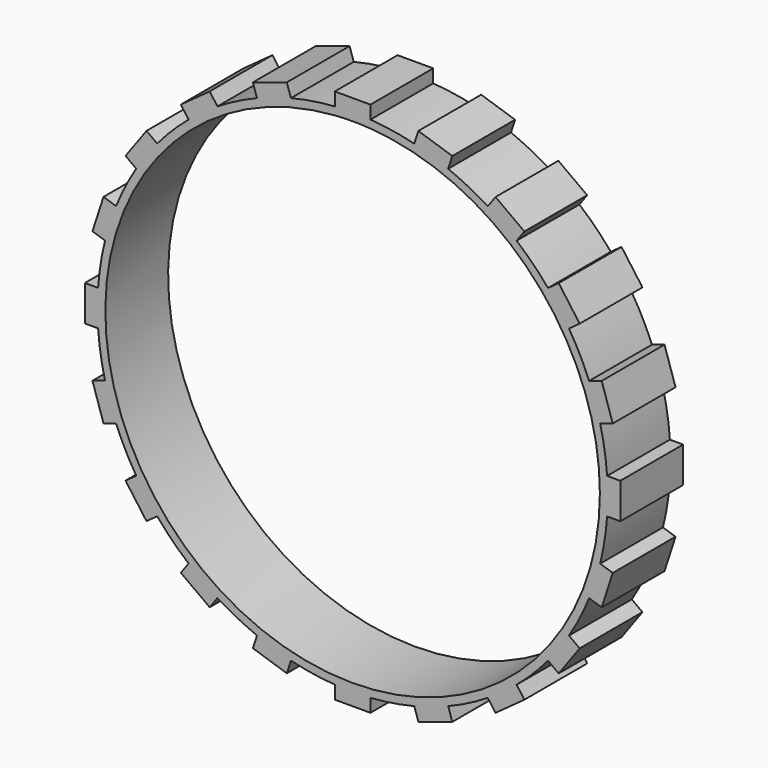
from build123d import *

# Parameters (mm, degrees)
F1_DEPTH = 10.16


with BuildPart() as f1:
    # F0 (on Front) → F1 (new body)
    with BuildSketch(Plane.XZ):
        with BuildLine():
            ThreePointArc((32.9392262703, -2.3081968538), (32.9998003891, -1.1548048657), (33.02, 0))
            ThreePointArc((33.02, 0), (32.9998003891, 1.1548048657), (32.9392262703, 2.3081968538))
            ThreePointArc((32.9392262703, 2.3081968538), (32.6134690065, 5.1654660356), (32.0403378403, 7.9835550403))
            ThreePointArc((32.0403378403, 7.9835550403), (31.4038861681, 10.2037411543), (30.6137937319, 12.3740063578))
            ThreePointArc((30.6137937319, 12.3740063578), (29.4210354287, 14.9907663014), (28.0051179043, 17.4938209425))
            ThreePointArc((28.0051179043, 17.4938209425), (26.7137411543, 19.4086690307), (25.2916697641, 21.2285619047))
            ThreePointArc((25.2916697641, 21.2285619047), (23.3486659148, 23.3486659148), (21.2285619047, 25.2916697641))
            ThreePointArc((21.2285619047, 25.2916697641), (19.4086690307, 26.7137411543), (17.4938209425, 28.0051179043))
            ThreePointArc((17.4938209425, 28.0051179043), (14.9907663014, 29.4210354287), (12.3740063578, 30.6137937319))
            ThreePointArc((12.3740063578, 30.6137937319), (10.2037411543, 31.4038861681), (7.9835550403, 32.0403378403))
            ThreePointArc((7.9835550403, 32.0403378403), (5.1654660356, 32.6134690065), (2.3081968538, 32.9392262703))
            ThreePointArc((2.3081968538, 32.9392262703), (0, 33.02), (-2.3081968538, 32.9392262703))
            ThreePointArc((-2.3081968538, 32.9392262703), (-5.1654660356, 32.6134690065), (-7.9835550403, 32.0403378403))
            ThreePointArc((-7.9835550403, 32.0403378403), (-10.2037411543, 31.4038861681), (-12.3740063578, 30.6137937319))
            ThreePointArc((-12.3740063578, 30.6137937319), (-14.9907663014, 29.4210354287), (-17.4938209425, 28.0051179043))
            ThreePointArc((-17.4938209425, 28.0051179043), (-19.4086690307, 26.7137411543), (-21.2285619047, 25.2916697641))
            ThreePointArc((-21.2285619047, 25.2916697641), (-23.3486659148, 23.3486659148), (-25.2916697641, 21.2285619047))
            ThreePointArc((-25.2916697641, 21.2285619047), (-26.7137411543, 19.4086690307), (-28.0051179043, 17.4938209425))
            ThreePointArc((-28.0051179043, 17.4938209425), (-29.4210354287, 14.9907663014), (-30.6137937319, 12.3740063578))
            ThreePointArc((-30.6137937319, 12.3740063578), (-31.4038861681, 10.2037411543), (-32.0403378403, 7.9835550403))
            ThreePointArc((-32.0403378403, 7.9835550403), (-32.6134690065, 5.1654660356), (-32.9392262703, 2.3081968538))
            ThreePointArc((-32.9392262703, 2.3081968538), (-33.02, 0), (-32.9392262703, -2.3081968538))
            ThreePointArc((-32.9392262703, -2.3081968538), (-32.6134690065, -5.1654660356), (-32.0403378403, -7.9835550403))
            ThreePointArc((-32.0403378403, -7.9835550403), (-31.4038861681, -10.2037411543), (-30.6137937319, -12.3740063578))
            ThreePointArc((-30.6137937319, -12.3740063578), (-29.4210354287, -14.9907663014), (-28.0051179043, -17.4938209425))
            ThreePointArc((-28.0051179043, -17.4938209425), (-26.7137411543, -19.4086690307), (-25.2916697641, -21.2285619047))
            ThreePointArc((-25.2916697641, -21.2285619047), (-23.3486659148, -23.3486659148), (-21.2285619047, -25.2916697641))
            ThreePointArc((-21.2285619047, -25.2916697641), (-19.4086690307, -26.7137411543), (-17.4938209425, -28.0051179043))
            ThreePointArc((-17.4938209425, -28.0051179043), (-14.9907663014, -29.4210354287), (-12.3740063578, -30.6137937319))
            ThreePointArc((-12.3740063578, -30.6137937319), (-10.2037411543, -31.4038861681), (-7.9835550403, -32.0403378403))
            ThreePointArc((-7.9835550403, -32.0403378403), (-5.1654660356, -32.6134690065), (-2.3081968538, -32.9392262703))
            ThreePointArc((-2.3081968538, -32.9392262703), (0, -33.02), (2.3081968538, -32.9392262703))
            ThreePointArc((2.3081968538, -32.9392262703), (5.1654660356, -32.6134690065), (7.9835550403, -32.0403378403))
            ThreePointArc((7.9835550403, -32.0403378403), (10.2037411543, -31.4038861681), (12.3740063578, -30.6137937319))
            ThreePointArc((12.3740063578, -30.6137937319), (14.9907663014, -29.4210354287), (17.4938209425, -28.0051179043))
            ThreePointArc((17.4938209425, -28.0051179043), (19.4086690307, -26.7137411543), (21.2285619047, -25.2916697641))
            ThreePointArc((21.2285619047, -25.2916697641), (23.3486659148, -23.3486659148), (25.2916697641, -21.2285619047))
            ThreePointArc((25.2916697641, -21.2285619047), (26.7137411543, -19.4086690307), (28.0051179043, -17.4938209425))
            ThreePointArc((28.0051179043, -17.4938209425), (29.4210354287, -14.9907663014), (30.6137937319, -12.3740063578))
            ThreePointArc((30.6137937319, -12.3740063578), (31.4038861681, -10.2037411543), (32.0403378403, -7.9835550403))
            ThreePointArc((32.0403378403, -7.9835550403), (32.6134690065, -5.1654660356), (32.9392262703, -2.3081968538))
        make_face()
        with BuildLine():
            ThreePointArc((2.3081968538, 31.9206554332), (23.4321098934, 21.7989046042), (32.004, 0))
            ThreePointArc((32.004, 0), (-21.7989046042, -23.4321098934), (-2.3081968538, 31.9206554332))
            ThreePointArc((-2.3081968538, 31.9206554332), (0, 32.004), (2.3081968538, 31.9206554332))
        make_face(mode=Mode.SUBTRACT)
        with BuildLine():
            ThreePointArc((32.9392262703, 2.3081968538), (32.9998003891, 1.1548048657), (33.02, 0))
            ThreePointArc((33.02, 0), (32.9998003891, -1.1548048657), (32.9392262703, -2.3081968538))
            Line((32.9392262703, -2.3081968538), (34.6495732665, -2.3081968538))
            Line((34.6495732665, -2.3081968538), (34.6495732665, 2.3081968538))
            Line((34.6495732665, 2.3081968538), (32.9392262703, 2.3081968538))
        make_face()
        with BuildLine():
            ThreePointArc((30.6137937319, 12.3740063578), (31.4038861681, 10.2037411543), (32.0403378403, 7.9835550403))
            Line((32.0403378403, 7.9835550403), (33.6669744962, 8.5120813284))
            Line((33.6669744962, 8.5120813284), (32.2404303878, 12.9025326459))
            Line((32.2404303878, 12.9025326459), (30.6137937319, 12.3740063578))
        make_face()
        with BuildLine():
            Line((33.6669744962, -8.5120813284), (32.0403378403, -7.9835550403))
            ThreePointArc((32.0403378403, -7.9835550403), (31.4038861681, -10.2037411543), (30.6137937319, -12.3740063578))
            Line((30.6137937319, -12.3740063578), (32.2404303878, -12.9025326459))
            Line((32.2404303878, -12.9025326459), (33.6669744962, -8.5120813284))
        make_face()
        with BuildLine():
            ThreePointArc((25.2916697641, 21.2285619047), (26.7137411543, 19.4086690307), (28.0051179043, 17.4938209425))
            Line((28.0051179043, 17.4938209425), (29.3888176905, 18.4991376832))
            Line((29.3888176905, 18.4991376832), (26.6753695504, 22.2338786454))
            Line((26.6753695504, 22.2338786454), (25.2916697641, 21.2285619047))
        make_face()
        with BuildLine():
            Line((29.3888176905, -18.4991376832), (28.0051179043, -17.4938209425))
            ThreePointArc((28.0051179043, -17.4938209425), (26.7137411543, -19.4086690307), (25.2916697641, -21.2285619047))
            Line((25.2916697641, -21.2285619047), (26.6753695504, -22.2338786454))
            Line((26.6753695504, -22.2338786454), (29.3888176905, -18.4991376832))
        make_face()
        with BuildLine():
            ThreePointArc((17.4938209425, 28.0051179043), (19.4086690307, 26.7137411543), (21.2285619047, 25.2916697641))
            Line((21.2285619047, 25.2916697641), (22.2338786454, 26.6753695504))
            Line((22.2338786454, 26.6753695504), (18.4991376832, 29.3888176905))
            Line((18.4991376832, 29.3888176905), (17.4938209425, 28.0051179043))
        make_face()
        with BuildLine():
            Line((22.2338786454, -26.6753695504), (21.2285619047, -25.2916697641))
            ThreePointArc((21.2285619047, -25.2916697641), (19.4086690307, -26.7137411543), (17.4938209425, -28.0051179043))
            Line((17.4938209425, -28.0051179043), (18.4991376832, -29.3888176905))
            Line((18.4991376832, -29.3888176905), (22.2338786454, -26.6753695504))
        make_face()
        with BuildLine():
            ThreePointArc((7.9835550403, 32.0403378403), (10.2037411543, 31.4038861681), (12.3740063578, 30.6137937319))
            Line((12.3740063578, 30.6137937319), (12.9025326459, 32.2404303878))
            Line((12.9025326459, 32.2404303878), (8.5120813284, 33.6669744962))
            Line((8.5120813284, 33.6669744962), (7.9835550403, 32.0403378403))
        make_face()
        with BuildLine():
            Line((12.9025326459, -32.2404303878), (12.3740063578, -30.6137937319))
            ThreePointArc((12.3740063578, -30.6137937319), (10.2037411543, -31.4038861681), (7.9835550403, -32.0403378403))
            Line((7.9835550403, -32.0403378403), (8.5120813284, -33.6669744962))
            Line((8.5120813284, -33.6669744962), (12.9025326459, -32.2404303878))
        make_face()
        with BuildLine():
            ThreePointArc((-2.3081968538, 32.9392262703), (0, 33.02), (2.3081968538, 32.9392262703))
            Line((2.3081968538, 32.9392262703), (2.3081968538, 34.6495732665))
            Line((2.3081968538, 34.6495732665), (-2.3081968538, 34.6495732665))
            Line((-2.3081968538, 34.6495732665), (-2.3081968538, 32.9392262703))
        make_face()
        with BuildLine():
            Line((2.3081968538, -34.6495732665), (2.3081968538, -32.9392262703))
            ThreePointArc((2.3081968538, -32.9392262703), (0, -33.02), (-2.3081968538, -32.9392262703))
            Line((-2.3081968538, -32.9392262703), (-2.3081968538, -34.6495732665))
            Line((-2.3081968538, -34.6495732665), (2.3081968538, -34.6495732665))
        make_face()
        with BuildLine():
            ThreePointArc((-12.3740063578, 30.6137937319), (-10.2037411543, 31.4038861681), (-7.9835550403, 32.0403378403))
            Line((-7.9835550403, 32.0403378403), (-8.5120813284, 33.6669744962))
            Line((-8.5120813284, 33.6669744962), (-12.9025326459, 32.2404303878))
            Line((-12.9025326459, 32.2404303878), (-12.3740063578, 30.6137937319))
        make_face()
        with BuildLine():
            Line((-8.5120813284, -33.6669744962), (-7.9835550403, -32.0403378403))
            ThreePointArc((-7.9835550403, -32.0403378403), (-10.2037411543, -31.4038861681), (-12.3740063578, -30.6137937319))
            Line((-12.3740063578, -30.6137937319), (-12.9025326459, -32.2404303878))
            Line((-12.9025326459, -32.2404303878), (-8.5120813284, -33.6669744962))
        make_face()
        with BuildLine():
            ThreePointArc((-21.2285619047, 25.2916697641), (-19.4086690307, 26.7137411543), (-17.4938209425, 28.0051179043))
            Line((-17.4938209425, 28.0051179043), (-18.4991376832, 29.3888176905))
            Line((-18.4991376832, 29.3888176905), (-22.2338786454, 26.6753695504))
            Line((-22.2338786454, 26.6753695504), (-21.2285619047, 25.2916697641))
        make_face()
        with BuildLine():
            Line((-18.4991376832, -29.3888176905), (-17.4938209425, -28.0051179043))
            ThreePointArc((-17.4938209425, -28.0051179043), (-19.4086690307, -26.7137411543), (-21.2285619047, -25.2916697641))
            Line((-21.2285619047, -25.2916697641), (-22.2338786454, -26.6753695504))
            Line((-22.2338786454, -26.6753695504), (-18.4991376832, -29.3888176905))
        make_face()
        with BuildLine():
            ThreePointArc((-28.0051179043, 17.4938209425), (-26.7137411543, 19.4086690307), (-25.2916697641, 21.2285619047))
            Line((-25.2916697641, 21.2285619047), (-26.6753695504, 22.2338786454))
            Line((-26.6753695504, 22.2338786454), (-29.3888176905, 18.4991376832))
            Line((-29.3888176905, 18.4991376832), (-28.0051179043, 17.4938209425))
        make_face()
        with BuildLine():
            Line((-26.6753695504, -22.2338786454), (-25.2916697641, -21.2285619047))
            ThreePointArc((-25.2916697641, -21.2285619047), (-26.7137411543, -19.4086690307), (-28.0051179043, -17.4938209425))
            Line((-28.0051179043, -17.4938209425), (-29.3888176905, -18.4991376832))
            Line((-29.3888176905, -18.4991376832), (-26.6753695504, -22.2338786454))
        make_face()
        with BuildLine():
            ThreePointArc((-32.0403378403, 7.9835550403), (-31.4038861681, 10.2037411543), (-30.6137937319, 12.3740063578))
            Line((-30.6137937319, 12.3740063578), (-32.2404303878, 12.9025326459))
            Line((-32.2404303878, 12.9025326459), (-33.6669744962, 8.5120813284))
            Line((-33.6669744962, 8.5120813284), (-32.0403378403, 7.9835550403))
        make_face()
        with BuildLine():
            Line((-32.2404303878, -12.9025326459), (-30.6137937319, -12.3740063578))
            ThreePointArc((-30.6137937319, -12.3740063578), (-31.4038861681, -10.2037411543), (-32.0403378403, -7.9835550403))
            Line((-32.0403378403, -7.9835550403), (-33.6669744962, -8.5120813284))
            Line((-33.6669744962, -8.5120813284), (-32.2404303878, -12.9025326459))
        make_face()
        with BuildLine():
            ThreePointArc((-32.9392262703, -2.3081968538), (-33.02, 0), (-32.9392262703, 2.3081968538))
            Line((-32.9392262703, 2.3081968538), (-34.6495732665, 2.3081968538))
            Line((-34.6495732665, 2.3081968538), (-34.6495732665, -2.3081968538))
            Line((-34.6495732665, -2.3081968538), (-32.9392262703, -2.3081968538))
        make_face()
    extrude(amount=F1_DEPTH)


solid = f1.part
